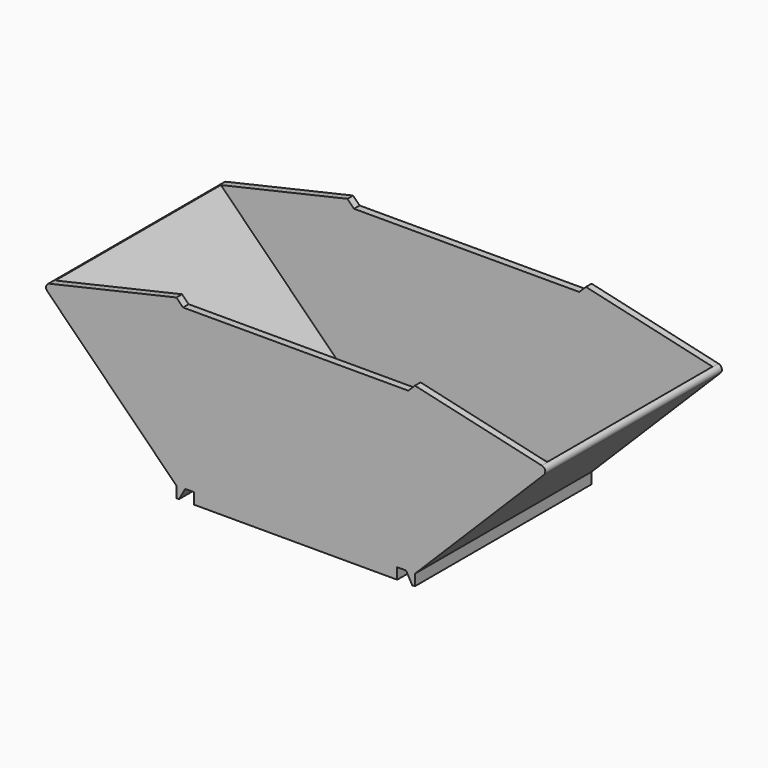
from build123d import *

# Parameters (mm, degrees)
F1_DEPTH        = 50
F2_T            = -3.2
F3_R            = 1
F4_DEPTH        = 5.001
F4_COPIES_COUNT = 8
F5_W            = 93.6
F5_H            = 50
F6_DEPTH        = 150
F7_R            = 2
F8_R            = 2


# Not quite as in the source:
# - a pattern or mirror of a feature is missing from the dataset's text; its kind, count and spacing are read off the source's solid
# - a feature names something its author has since deleted; it is built from what else it names


with BuildPart() as f1:
    # F0 (on Front) → F1 (new body, symmetric)
    with BuildSketch(Plane.XZ):
        Polygon((-52.8, -5), (-50, 0), (-46, 0), (-46, -5), (46, -5), (46, 0), (50, 0), (52.8, -5), (54, -5), (54, 0), (115, 61), (54, 75), (51, 72), (-51, 72), (-54, 75), (-115, 61), (-54, 0), (-54, -5), align=None)
    extrude(amount=F1_DEPTH, both=True)

    # F2
    f2_openings = [f1.faces().sort_by_distance(p)[0] for p in [
        (-84.5, 0, 68),
        (84.5, 0, 68),
    ]]
    offset(amount=F2_T, openings=f2_openings, kind=Kind.INTERSECTION)

    # F3 (on Top) → F4 (cut, through all)
    with BuildSketch(Plane.XY):
        with Locations((-3.2352380638, -12.0740728286)):
            Circle(F3_R)
    f4 = extrude(amount=-F4_DEPTH, mode=Mode.SUBTRACT)

    # F4_copies: F4 ×8 about axis
    f4_copies_axis = Axis((0, 0, 0), (0, 0, 1))
    for i in range(1, F4_COPIES_COUNT):
        add(f4.rotate(f4_copies_axis, i * 360 / F4_COPIES_COUNT), mode=Mode.SUBTRACT)

    # F5 (on Right) → F6 (cut, symmetric)
    with BuildSketch(Plane.YZ):
        with Locations((0, 90)):
            Rectangle(F5_W, F5_H)
    extrude(amount=F6_DEPTH, both=True, mode=Mode.SUBTRACT)

    # F7
    f7_edges = [f1.edges().sort_by_distance(p)[0] for p in [
        (115, 0, 61),
        (-115, 0, 61),
    ]]
    fillet(f7_edges, radius=F7_R)

    # F8
    f8_edges = [f1.edges().sort_by_distance(p)[0] for p in [
        (42.8, 0, -1.8),
        (0, -46.8, -1.8),
        (0, 46.8, -1.8),
        (-42.8, 0, -1.8),
        (-5.542893, 11.532424, -1.8),
        (-12.074073, 4.235238, -1.8),
        (4.235238, 12.074073, -1.8),
        (11.532424, 5.542893, -1.8),
        (-11.532424, -5.542893, -1.8),
        (-4.235238, -12.074073, -1.8),
        (12.074073, -4.235238, -1.8),
        (5.542893, -11.532424, -1.8),
    ]]
    fillet(f8_edges, radius=F8_R)


solid = f1.part
